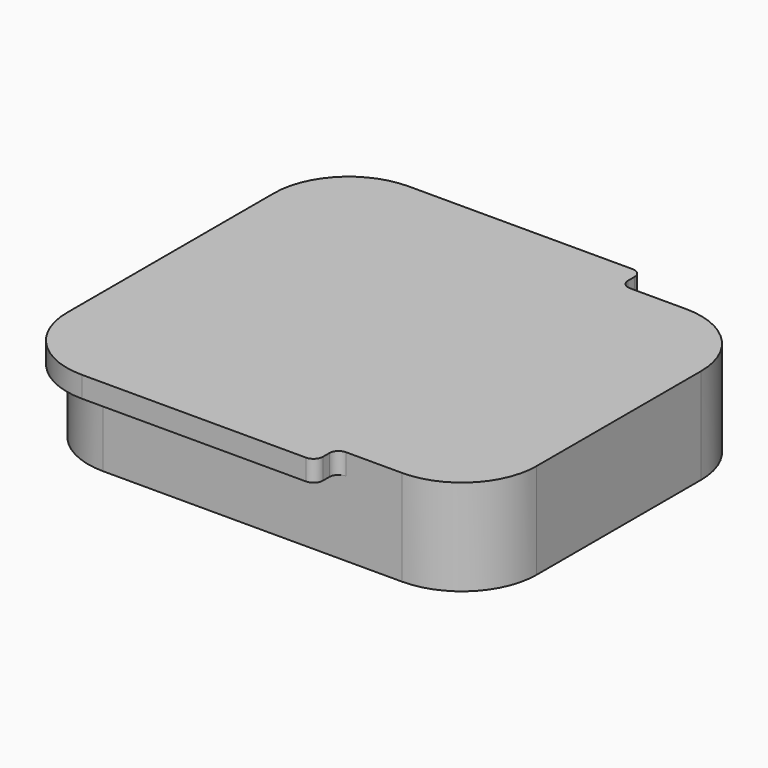
from build123d import *

# Parameters (mm, degrees)
F1_DEPTH     = 10.25
F3_DEPTH     = 2.25
F4_R         = 1
F5_T         = 1.9
F5_T3_DEPTH  = 4.8
F5_T5_DEPTH  = 28.8
F5_T8_ANGLE  = 90.000000001
F5_T10_ANGLE = 90.000000001


# Not quite as in the source:
# - a shell that OpenCascade refuses in one call is made with other operations: the cavity is built on its own and cut out


with BuildPart() as f1:
    # F0 (on Top) → F1 (new body)
    with BuildSketch(Plane.XY):
        with BuildLine():
            ThreePointArc((24, 11), (21.6568542495, 16.6568542495), (16, 19))
            Line((16, 19), (-16, 19))
            ThreePointArc((-16, 19), (-21.6568542495, 16.6568542495), (-24, 11))
            Line((-24, 11), (-24, -11))
            ThreePointArc((-24, -11), (-21.6568542495, -16.6568542495), (-16, -19))
            Line((-16, -19), (16, -19))
            ThreePointArc((16, -19), (21.6568542495, -16.6568542495), (24, -11))
            Line((24, -11), (24, 11))
        make_face()
    extrude(amount=F1_DEPTH)

    # F2 (on face) → F3 (join)
    with BuildSketch(Plane.XY.offset(10.25)):
        with BuildLine():
            Line((8, 21.85), (-16, 21.85))
            ThreePointArc((-16, 21.85), (-21.6568542495, 19.5068542495), (-24, 13.85))
            Line((-24, 13.85), (-24, -13.85))
            ThreePointArc((-24, -13.85), (-21.6568542495, -19.5068542495), (-16, -21.85))
            Line((-16, -21.85), (8, -21.85))
            ThreePointArc((8, -21.85), (8.7071067812, -21.5571067812), (9, -20.85))
            Line((9, -20.85), (9, 20.85))
            ThreePointArc((9, 20.85), (8.7071067812, 21.5571067812), (8, 21.85))
        make_face()
    extrude(amount=-F3_DEPTH)

    # F4
    f4_edges = [f1.edges().sort_by_distance(p)[0] for p in [
        (9, -19, 9.125),
        (9, 19, 9.125),
    ]]
    fillet(f4_edges, radius=F4_R)

    # F5: shell of thickness 1.9, made by hand


with BuildPart() as f5_core1:
    # F5_t2: copy of F1
    add(f1.part)

    # the walls: a layer under each face that stays
    f5_faces = [f5_core1.faces().sort_by_distance(p)[0] for p in [
        (0, 0, 10.25),
        (0, 19, 5.125),
        (9.2928932188, 19.2928932188, 9.125),
        (21.6568542495, 16.6568542495, 5.125),
        (9, 20.425, 9.125),
        (24, 0, 5.125),
        (21.6568542495, -16.6568542495, 5.125),
        (-4, 21.85, 9.125),
        (0, -19, 5.125),
        (-21.6568542495, 19.5068542495, 9.125),
        (9.2928932188, -19.2928932188, 9.125),
        (-24, 0, 5.125),
        (9, -20.425, 9.125),
        (-21.6568542495, -19.5068542495, 9.125),
        (-4, -21.85, 9.125),
        (-18.3333333333, 20.0416666667, 8),
        (-21.6568542495, 16.6568542495, 4),
        (-18.3333333333, -20.0416666667, 8),
        (-21.6568542495, -16.6568542495, 4),
    ]]
    thicken(f5_faces, amount=-F5_T, mode=Mode.SUBTRACT)

    # F5_s4 → F5_t3 (cut)
    with BuildSketch(Plane.YZ.offset(7.1)):
        Polygon((19.019, 7.981), (17.1, 8), (17.1, 9.9), (19, 9.9), align=None)
        Polygon((-19.019, 7.981), (-17.1, 8), (-17.1, 9.9), (-19, 9.9), align=None)
    extrude(amount=F5_T3_DEPTH, mode=Mode.SUBTRACT)

    # F5_s6 → F5_t5 (cut)
    with BuildSketch(Plane.YZ.offset(-17.9)):
        Polygon((19.019, 7.981), (17.1, 8), (17.1, 9.9), (19, 9.9), align=None)
        Polygon((-19.019, 7.981), (-17.1, 8), (-17.1, 9.9), (-19, 9.9), align=None)
    extrude(amount=F5_T5_DEPTH, mode=Mode.SUBTRACT)

    # F5_s7 → F5_t8 (revolve, cut)
    with BuildSketch(Plane.XZ.offset(-11)):
        Polygon((-24.019, 7.981), (-24, 9.9), (-22.1, 9.9), (-22.1, 8), align=None)
    revolve(axis=Axis((-16, 11, 8), (0, 0, -1)), revolution_arc=F5_T8_ANGLE, mode=Mode.SUBTRACT)

    # F5_s9 → F5_t10 (revolve, cut)
    with BuildSketch(Plane.YZ.offset(-16)):
        Polygon((-19.019, 7.981), (-19, 9.9), (-17.1, 9.9), (-17.1, 8), align=None)
    revolve(axis=Axis((-16, -11, 8), (0, 0, -1)), revolution_arc=F5_T10_ANGLE, mode=Mode.SUBTRACT)


with BuildPart() as f1_1:
    add(f1.part)

    # what is left inside the walls is the cavity
    f5_cavity = [f5_core1.part.solids().sort_by_distance(p)[0] for p in [
        (0, -5.7, 8.331),
    ]]
    add(f5_cavity, mode=Mode.SUBTRACT)


solid = f1_1.part
